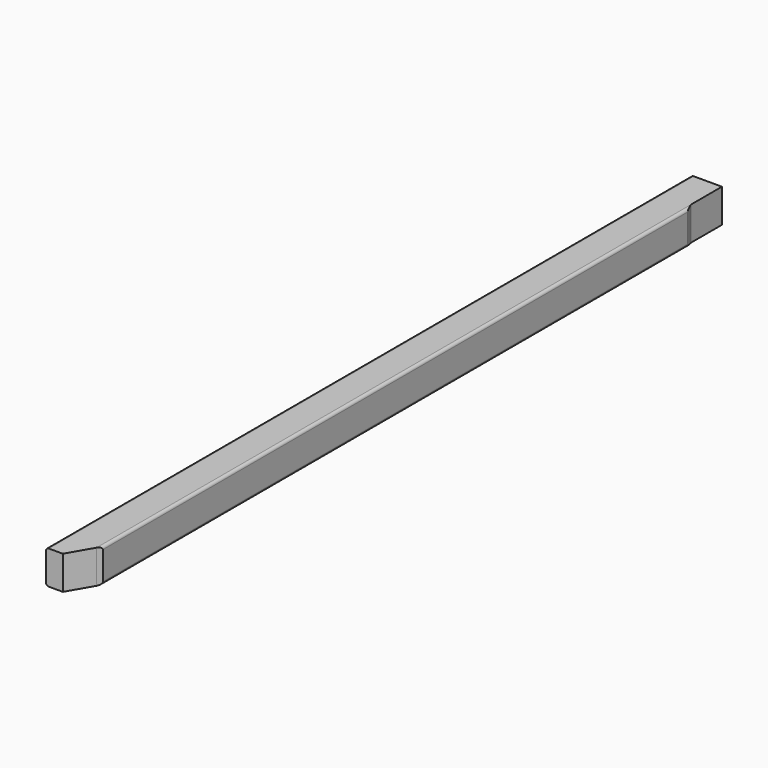
from build123d import *

# Parameters (mm, degrees)
F1_DEPTH = 600
F3_DEPTH = 25.001


with BuildPart() as f1:
    # F0 (on Front) → F1 (new body)
    with BuildSketch(Plane.XZ):
        with BuildLine():
            ThreePointArc((12.5, 10.5), (11.9142135624, 11.9142135624), (10.5, 12.5))
            Line((10.5, 12.5), (-10.5, 12.5))
            ThreePointArc((-10.5, 12.5), (-11.9142135624, 11.9142135624), (-12.5, 10.5))
            Line((-12.5, 10.5), (-12.5, -10.5))
            ThreePointArc((-12.5, -10.5), (-11.9142135624, -11.9142135624), (-10.5, -12.5))
            Line((-10.5, -12.5), (10.5, -12.5))
            ThreePointArc((10.5, -12.5), (11.9142135624, -11.9142135624), (12.5, -10.5))
            Line((12.5, -10.5), (12.5, 10.5))
        make_face()
    extrude(amount=F1_DEPTH)

    # F2 (on face) → F3 (cut, through all)
    with BuildSketch(Plane.XY.offset(12.5)):
        Polygon((12.5, -34.3434677432), (12.5, 0), (10.5, 0), (10.5, -28.8485129043), align=None)
        Polygon((10.5, -600), (10.5, -581.8134665205), (0, -600), align=None)
        Polygon((12.5, -578.3493649054), (10.5, -581.8134665205), (10.5, -600), (12.5, -600), align=None)
    extrude(amount=-F3_DEPTH, mode=Mode.SUBTRACT)


solid = f1.part
